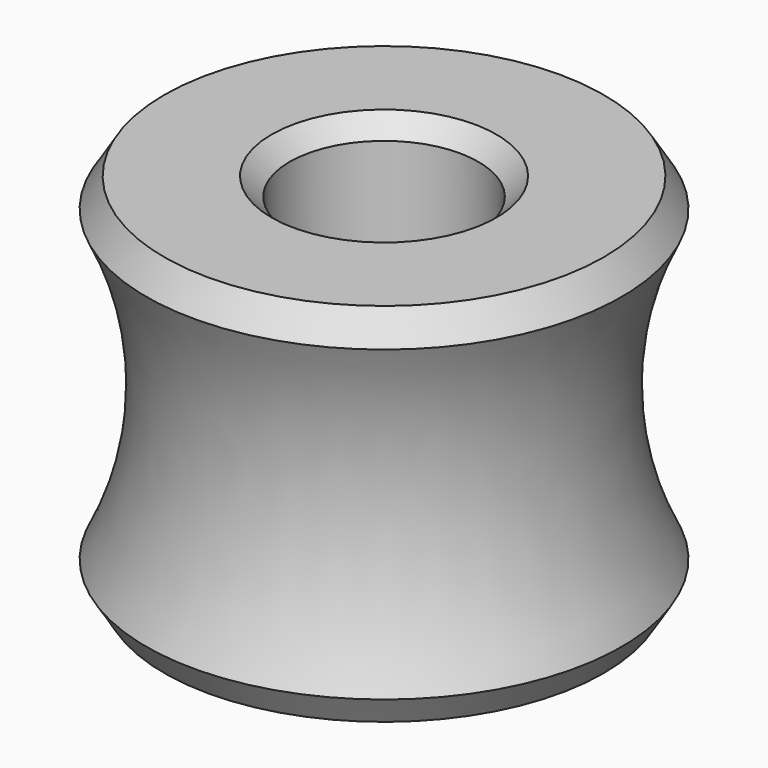
from build123d import *

# Parameters (mm, degrees)
F2_SIZE = 1


# Not quite as in the source:
# - a fillet or chamfer that OpenCascade refuses, or shapes differently, is made with other operations: its cross-section is extruded or revolved along the edge and cut away or added


with BuildPart() as f1:
    # F0 (on Front) → F1 (revolve)
    with BuildSketch(Plane.XZ):
        with BuildLine():
            Line((-5.2, 0), (-5.2, 20.18))
            Line((-5.2, 20.18), (-14, 20.18))
            ThreePointArc((-14, 20.18), (-11.0994378784, 10.09), (-14, 0))
            Line((-14, 0), (-5.2, 0))
        make_face()
    revolve(axis=Axis((0, 0, 10.09), (0, 0, 1)))

    # F2
    f2_edges = [f1.edges().sort_by_distance(p)[0] for p in [
        (5.2, 0, 0),
        (5.2, 0, 20.18),
        (-5.2, 0, 10.09),
    ]]
    chamfer(f2_edges, length=F2_SIZE)

    # F3: chamfer of 2 on 3 edges, made by hand

    # F3_s1 → F3_t2 (revolve, cut)
    with BuildSketch(Plane.XZ):
        with BuildLine():
            Line((-13.1431767576, 18.5105716839), (-12.0687646644, 20.2480416136))
            Line((-12.0687646644, 20.2480416136), (-12.0687646644, 20.2880416136))
            ThreePointArc((-12.0687646644, 20.2880416136), (-13.0343823322, 20.22), (-14, 20.22))
            Line((-14, 20.22), (-14.0338935534, 20.1587578947))
            ThreePointArc((-14.0338935534, 20.1587578947), (-13.556591594, 19.3536837603), (-13.1789627292, 18.4927009191))
            Line((-13.1789627292, 18.4927009191), (-13.1431767576, 18.5105716839))
        make_face()
    revolve(axis=Axis((0, 0, 20.18), (0, 0, 1)), mode=Mode.SUBTRACT)

    # F3_s3 → F3_t4 (revolve, cut)
    with BuildSketch(Plane.XZ):
        with BuildLine():
            Line((-12.0687646644, -0.0680416136), (-13.1431767576, 1.6694283161))
            Line((-13.1431767576, 1.6694283161), (-13.1789627292, 1.6872990809))
            ThreePointArc((-13.1789627292, 1.6872990809), (-13.556591594, 0.8263162397), (-14.0338935534, 0.0212421053))
            Line((-14.0338935534, 0.0212421053), (-14, -0.04))
            ThreePointArc((-14, -0.04), (-13.0343823322, -0.04), (-12.0687646644, -0.1080416136))
            Line((-12.0687646644, -0.1080416136), (-12.0687646644, -0.0680416136))
        make_face()
    revolve(axis=Axis((0, 0, 0), (0, 0, 1)), mode=Mode.SUBTRACT)


solid = f1.part
